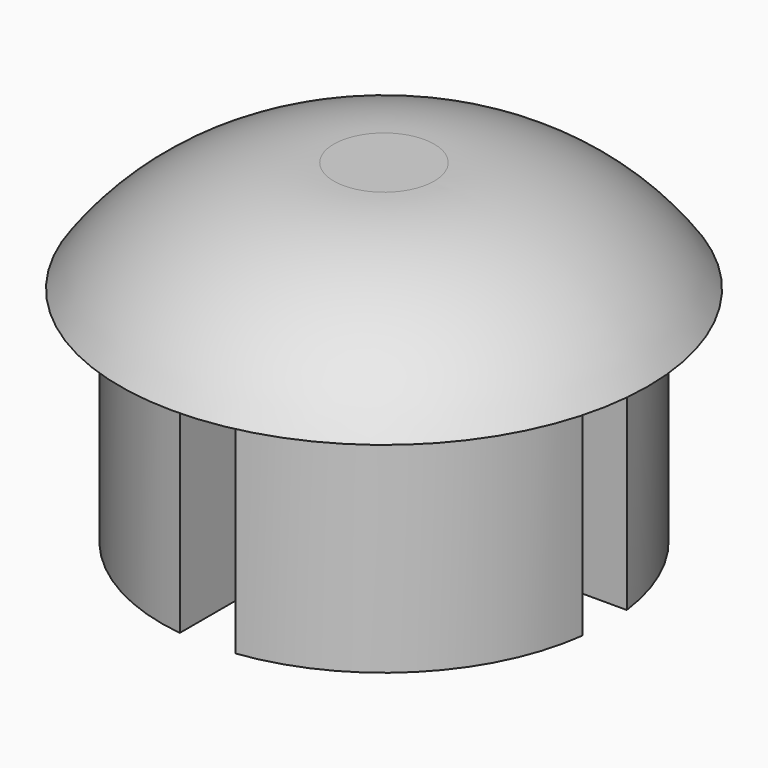
from build123d import *

# Parameters (mm, degrees)
F0_R     = 4.75
F1_DEPTH = 2
F2_DEPTH = 4


# Not quite as in the source:
# - a fillet or chamfer that OpenCascade refuses, or shapes differently, is made with other operations: its cross-section is extruded or revolved along the edge and cut away or added
# - a feature names something its author has since deleted; it is built from what else it names


with BuildPart() as f1:
    # F0 (on Top) → F1 (new body)
    with BuildSketch(Plane.XY):
        Circle(F0_R)
        with BuildLine():
            ThreePointArc((-0.5, -3.9686269666), (-2.8284271247, -2.8284271247), (-3.9686269666, -0.5))
            Line((-3.9686269666, -0.5), (-2.7549954628, -0.5))
            Line((-2.7549954628, -0.5), (-0.5, -0.5))
            Line((-0.5, -0.5), (-0.5, -2.7549954628))
            Line((-0.5, -2.7549954628), (-0.5, -3.9686269666))
        make_face(mode=Mode.SUBTRACT)
        with BuildLine():
            Line((0.5, -0.5), (2.7549954628, -0.5))
            Line((2.7549954628, -0.5), (3.9686269666, -0.5))
            ThreePointArc((3.9686269666, -0.5), (2.8284271247, -2.8284271247), (0.5, -3.9686269666))
            Line((0.5, -3.9686269666), (0.5, -2.7549954628))
            Line((0.5, -2.7549954628), (0.5, -0.5))
        make_face(mode=Mode.SUBTRACT)
        with BuildLine():
            Line((-2.7549954628, 0.5), (-3.9686269666, 0.5))
            ThreePointArc((-3.9686269666, 0.5), (-2.8284271247, 2.8284271247), (-0.5, 3.9686269666))
            Line((-0.5, 3.9686269666), (-0.5, 2.7549954628))
            Line((-0.5, 2.7549954628), (-0.5, 0.5))
            Line((-0.5, 0.5), (-2.7549954628, 0.5))
        make_face(mode=Mode.SUBTRACT)
        with BuildLine():
            Line((3.9686269666, 0.5), (2.7549954628, 0.5))
            Line((2.7549954628, 0.5), (0.5, 0.5))
            Line((0.5, 0.5), (0.5, 2.7549954628))
            Line((0.5, 2.7549954628), (0.5, 3.9686269666))
            ThreePointArc((0.5, 3.9686269666), (2.8284271247, 2.8284271247), (3.9686269666, 0.5))
        make_face(mode=Mode.SUBTRACT)
        with BuildLine():
            Line((-2.7549954628, -0.5), (-3.9686269666, -0.5))
            ThreePointArc((-3.9686269666, -0.5), (-2.8284271247, -2.8284271247), (-0.5, -3.9686269666))
            Line((-0.5, -3.9686269666), (-0.5, -2.7549954628))
            Line((-0.5, -2.7549954628), (-0.5, -0.5))
            Line((-0.5, -0.5), (-2.7549954628, -0.5))
        make_face()
        with BuildLine():
            ThreePointArc((-0.5, 3.9686269666), (-2.8284271247, 2.8284271247), (-3.9686269666, 0.5))
            Line((-3.9686269666, 0.5), (-2.7549954628, 0.5))
            Line((-2.7549954628, 0.5), (-0.5, 0.5))
            Line((-0.5, 0.5), (-0.5, 2.7549954628))
            Line((-0.5, 2.7549954628), (-0.5, 3.9686269666))
        make_face()
        with BuildLine():
            Line((0.5, 0.5), (2.7549954628, 0.5))
            Line((2.7549954628, 0.5), (3.9686269666, 0.5))
            ThreePointArc((3.9686269666, 0.5), (2.8284271247, 2.8284271247), (0.5, 3.9686269666))
            Line((0.5, 3.9686269666), (0.5, 2.7549954628))
            Line((0.5, 2.7549954628), (0.5, 0.5))
        make_face()
        with BuildLine():
            Line((3.9686269666, -0.5), (2.7549954628, -0.5))
            Line((2.7549954628, -0.5), (0.5, -0.5))
            Line((0.5, -0.5), (0.5, -2.7549954628))
            Line((0.5, -2.7549954628), (0.5, -3.9686269666))
            ThreePointArc((0.5, -3.9686269666), (2.8284271247, -2.8284271247), (3.9686269666, -0.5))
        make_face()
    extrude(amount=F1_DEPTH)

    # F0 (on Top) → F2 (join)
    with BuildSketch(Plane.XY):
        with BuildLine():
            ThreePointArc((-0.5, 3.9686269666), (-2.8284271247, 2.8284271247), (-3.9686269666, 0.5))
            Line((-3.9686269666, 0.5), (-2.7549954628, 0.5))
            Line((-2.7549954628, 0.5), (-0.5, 0.5))
            Line((-0.5, 0.5), (-0.5, 2.7549954628))
            Line((-0.5, 2.7549954628), (-0.5, 3.9686269666))
        make_face()
        with BuildLine():
            Line((-2.7549954628, -0.5), (-3.9686269666, -0.5))
            ThreePointArc((-3.9686269666, -0.5), (-2.8284271247, -2.8284271247), (-0.5, -3.9686269666))
            Line((-0.5, -3.9686269666), (-0.5, -2.7549954628))
            Line((-0.5, -2.7549954628), (-0.5, -0.5))
            Line((-0.5, -0.5), (-2.7549954628, -0.5))
        make_face()
        with BuildLine():
            Line((3.9686269666, -0.5), (2.7549954628, -0.5))
            Line((2.7549954628, -0.5), (0.5, -0.5))
            Line((0.5, -0.5), (0.5, -2.7549954628))
            Line((0.5, -2.7549954628), (0.5, -3.9686269666))
            ThreePointArc((0.5, -3.9686269666), (2.8284271247, -2.8284271247), (3.9686269666, -0.5))
        make_face()
        with BuildLine():
            Line((0.5, 0.5), (2.7549954628, 0.5))
            Line((2.7549954628, 0.5), (3.9686269666, 0.5))
            ThreePointArc((3.9686269666, 0.5), (2.8284271247, 2.8284271247), (0.5, 3.9686269666))
            Line((0.5, 3.9686269666), (0.5, 2.7549954628))
            Line((0.5, 2.7549954628), (0.5, 0.5))
        make_face()
    extrude(amount=-F2_DEPTH)

    # F3: fillet of radius 4.7 on 1 edges, made by hand

    # F3_s1 → F3_t2 (revolve, cut)
    with BuildSketch(Plane.XZ):
        with BuildLine():
            ThreePointArc((4.75, 0), (3.0708715265, 1.4701318924), (0.9029231877, 2))
            Line((0.9029231877, 2), (4.75, 2))
            Line((4.75, 2), (4.75, 0))
        make_face()
    revolve(axis=Axis((0, 0, 2), (0, 0, 1)), mode=Mode.SUBTRACT)


solid = f1.part
